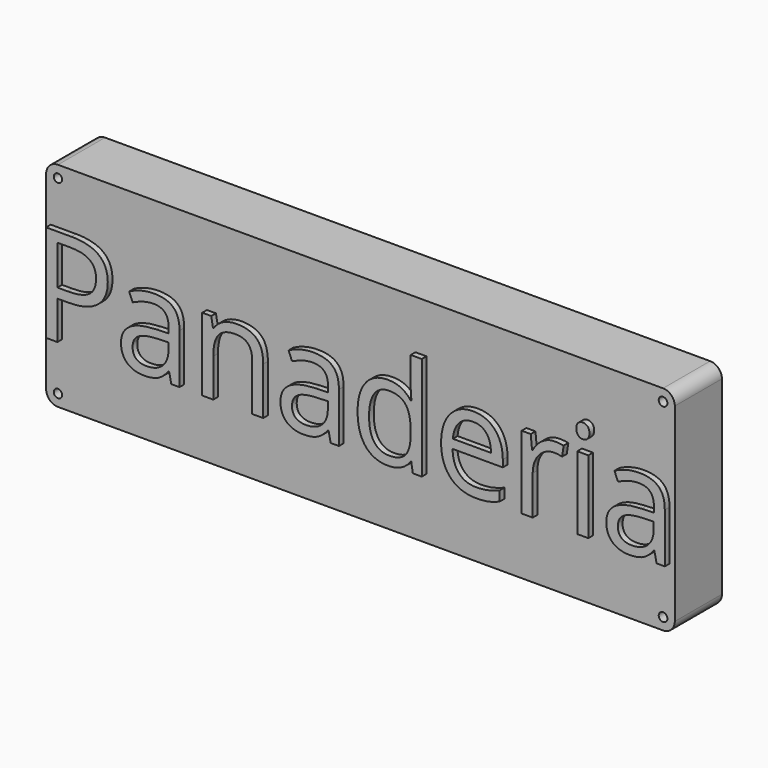
from build123d import *

# Parameters (mm, degrees)
F0_W         = 271.2024305947
F0_H         = 91.9632464647
F1_DEPTH     = 25.4
F2_TEXT_SIZE = 58.7882267104
F3_DEPTH     = 2.54
F4_R         = 5.08
F5_R         = 5.08
F6_R         = 5.08
F7_R         = 1.871733958
F7_R_2       = 1.7976772306
F8_DEPTH     = 36.83


# Not quite as in the source:
# - Text() gives the source's letters only with a copy of the font that has no kerning and outlines rounded to 1/6400 em; it was checked with that copy


with BuildPart() as f1:
    # F0 (on Front) → F1 (new body)
    with BuildSketch(Plane.XZ):
        with Locations((3.0390394386, 0)):
            Rectangle(F0_W, F0_H)
    extrude(amount=F1_DEPTH)

    # F2 (on face) → F3 (join)
    with BuildSketch(Plane.XZ.offset(25.4)):
        with Locations((-136.330679059, -19.732424058)):
            Text('Panaderia', F2_TEXT_SIZE, font='Open Sans', text_align=(TextAlign.LEFT, TextAlign.BOTTOM))
    extrude(amount=F3_DEPTH)

    # F4
    f4_edges = [f1.edges().sort_by_distance(p)[0] for p in [
        (138.640255, -12.7, 45.981623),
    ]]
    fillet(f4_edges, radius=F4_R)

    # F5
    f5_edges = [f1.edges().sort_by_distance(p)[0] for p in [
        (138.640255, -12.7, -45.981623),
    ]]
    fillet(f5_edges, radius=F5_R)

    # F6
    f6_edges = [f1.edges().sort_by_distance(p)[0] for p in [
        (-132.562176, -12.7, 45.981623),
        (-132.562176, -12.7, -45.981623),
    ]]
    fillet(f6_edges, radius=F6_R)

    # F7 (on face) → F8 (cut)
    with BuildSketch(Plane.XZ.offset(25.4)):
        with Locations((133.5602547359, 40.9016232324)):
            Circle(F7_R)
        with Locations((133.5602547359, -40.9016232324)):
            Circle(F7_R)
        with Locations((-127.4821758588, -40.9016232324)):
            Circle(F7_R_2)
        with Locations((-127.4821758588, 40.9016232324)):
            Circle(F7_R_2)
    extrude(amount=-F8_DEPTH, mode=Mode.SUBTRACT)


solid = f1.part
